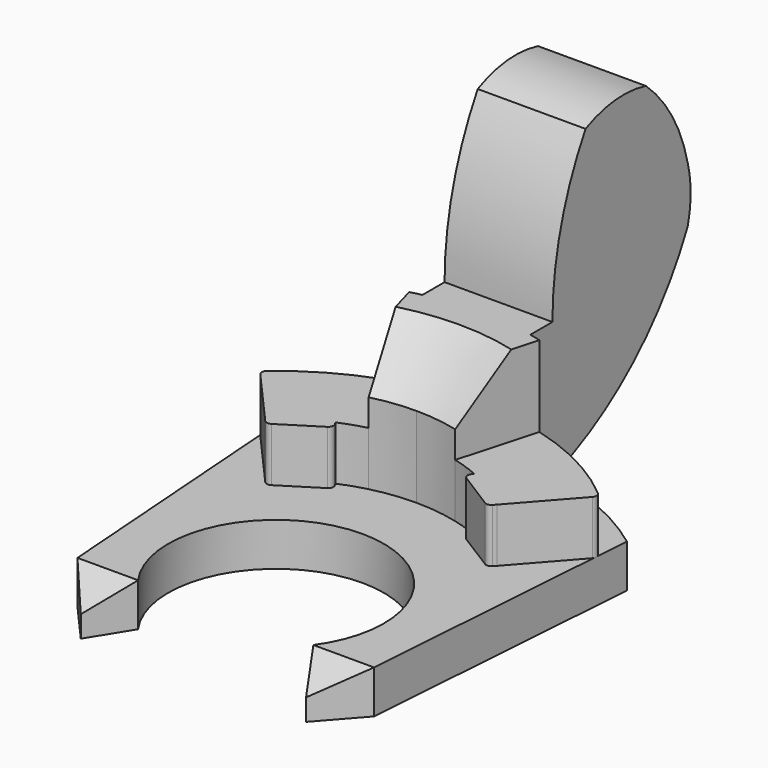
from build123d import *

# Parameters (mm, degrees)
F1_DEPTH      = 1.2
F1_DEPTH_BACK = 0.4
F3_DEPTH      = 12.5
F5_DEPTH      = 2
F6_DEPTH      = 5
F7_T2_ANGLE   = 119.2786087223
F8_DEPTH      = 5
F10_DEPTH     = 4
F11_DEPTH     = 5


# Not quite as in the source:
# - a fillet or chamfer that OpenCascade refuses, or shapes differently, is made with other operations: its cross-section is extruded or revolved along the edge and cut away or added
# - a feature names something its author has since deleted; it is built from what else it names


with BuildPart() as f1:
    # F0 (on Top) → F1 (new body, two sides)
    with BuildSketch(Plane.XY) as f1_sk:
        with BuildLine():
            ThreePointArc((-3.25, -2.3318447633), (0, 4), (3.25, -2.3318447633))
            Line((3.25, -2.3318447633), (4.1771243445, -3.8318447633))
            Line((4.1771243445, -3.8318447633), (5.5, -2.3318447633))
            Line((5.5, -2.3318447633), (6.2861850371, 8.4103434936))
            ThreePointArc((6.2861850371, 8.4103434936), (0, 10.5), (-6.2861850371, 8.4103434936))
            Line((-6.2861850371, 8.4103434936), (-5.5, -2.3318447633))
            Line((-5.5, -2.3318447633), (-4.1771243445, -3.8318447633))
            Line((-4.1771243445, -3.8318447633), (-3.25, -2.3318447633))
        make_face()
    extrude(amount=F1_DEPTH)
    extrude(f1_sk.sketch, amount=-F1_DEPTH_BACK)

    # F2 (on Right) → F3 (cut, symmetric)
    with BuildSketch(Plane.YZ):
        Polygon((-3.8318447633, 0.4), (-2.3318447633, 1.2), (-3.8318447633, 1.2), align=None)
    extrude(amount=F3_DEPTH, both=True, mode=Mode.SUBTRACT)

    # F4 (on face) → F5 (join)
    with BuildSketch(Plane.XY.offset(1.2)):
        with BuildLine():
            Line((0, 9.4893432962), (0, 9.5))
            ThreePointArc((0, 9.5), (-1.0056504861, 9.4466219941), (-2, 9.2870878105))
            ThreePointArc((-2, 9.2870878105), (-2.207287093, 9.2400153511), (-2.4134691055, 9.1883168686))
            Line((-2.4134691055, 9.1883168686), (-1.6054997382, 6.2986006851))
            ThreePointArc((-1.6054997382, 6.2986006851), (-0.809041268, 6.4494536378), (0, 6.5))
            Line((0, 6.5), (0, 9.4893432962))
        make_face()
        with BuildLine():
            Line((0, 10.3126084432), (0, 9.5))
            ThreePointArc((0, 9.5), (1.0056504861, 9.4466219941), (2, 9.2870878105))
            Line((2, 9.2870878105), (2, 10.3126084432))
            Line((2, 10.3126084432), (0, 10.3126084432))
        make_face()
        with BuildLine():
            ThreePointArc((2, 9.2870878105), (1.0056504861, 9.4466219941), (0, 9.5))
            Line((0, 9.5), (0, 9.4893432962))
            Line((0, 9.4893432962), (0, 6.5))
            ThreePointArc((0, 6.5), (0.809041268, 6.4494536378), (1.6054997382, 6.2986006851))
            Line((1.6054997382, 6.2986006851), (2.4134691055, 9.1883168686))
            ThreePointArc((2.4134691055, 9.1883168686), (2.207287093, 9.2400153511), (2, 9.2870878105))
        make_face()
        with BuildLine():
            ThreePointArc((-2, 9.2870878105), (-1.0056504861, 9.4466219941), (0, 9.5))
            Line((0, 9.5), (0, 10.3126084432))
            Line((0, 10.3126084432), (-2, 10.3126084432))
            Line((-2, 10.3126084432), (-2, 9.2870878105))
        make_face()
        with BuildLine():
            Line((-1.6054997382, 6.2986006851), (-2.4134691055, 9.1883168686))
            ThreePointArc((-2.4134691055, 9.1883168686), (-4.3834961594, 8.4282240965), (-6.1369591907, 7.2517399217))
            ThreePointArc((-6.1369591907, 7.2517399217), (-6.2072372931, 7.1135226449), (-6.1576144754, 6.9666192642))
            Line((-6.1576144754, 6.9666192642), (-4.3047045796, 4.8702688306))
            Line((-4.3047045796, 4.8702688306), (-4.2185888433, 4.7728389657))
            ThreePointArc((-4.2185888433, 4.7728389657), (-4.0971505607, 4.7073203992), (-3.9621862374, 4.7360357341))
            Line((-3.9621862374, 4.7360357341), (-2.5827247856, 5.6044208159))
            ThreePointArc((-2.5827247856, 5.6044208159), (-2.4942501859, 5.7293355978), (-2.5200172859, 5.8802246764))
            Line((-2.5200172859, 5.8802246764), (-2.5753119947, 5.968062343))
            ThreePointArc((-2.5753119947, 5.968062343), (-2.096928846, 6.152470188), (-1.6054997382, 6.2986006851))
        make_face()
        with BuildLine():
            ThreePointArc((6.1369591907, 7.2517399217), (4.3834961594, 8.4282240965), (2.4134691055, 9.1883168686))
            Line((2.4134691055, 9.1883168686), (1.6054997382, 6.2986006851))
            ThreePointArc((1.6054997382, 6.2986006851), (2.096928846, 6.152470188), (2.5753119947, 5.968062343))
            Line((2.5753119947, 5.968062343), (2.5200172859, 5.8802246764))
            ThreePointArc((2.5200172859, 5.8802246764), (2.4942501859, 5.7293355978), (2.5827247856, 5.6044208159))
            Line((2.5827247856, 5.6044208159), (3.9621862374, 4.7360357341))
            ThreePointArc((3.9621862374, 4.7360357341), (4.0971505607, 4.7073203992), (4.2185888433, 4.7728389657))
            Line((4.2185888433, 4.7728389657), (4.3047045796, 4.8702688306))
            Line((4.3047045796, 4.8702688306), (6.1576144754, 6.9666192642))
            ThreePointArc((6.1576144754, 6.9666192642), (6.2072372931, 7.1135226449), (6.1369591907, 7.2517399217))
        make_face()
    extrude(amount=F5_DEPTH)

    # F4 (on face) → F6 (join)
    with BuildSketch(Plane.XY.offset(1.2)):
        with BuildLine():
            ThreePointArc((2, 9.2870878105), (1.0056504861, 9.4466219941), (0, 9.5))
            Line((0, 9.5), (0, 9.4893432962))
            Line((0, 9.4893432962), (0, 6.5))
            ThreePointArc((0, 6.5), (0.809041268, 6.4494536378), (1.6054997382, 6.2986006851))
            Line((1.6054997382, 6.2986006851), (2.4134691055, 9.1883168686))
            ThreePointArc((2.4134691055, 9.1883168686), (2.207287093, 9.2400153511), (2, 9.2870878105))
        make_face()
        with BuildLine():
            Line((0, 9.4893432962), (0, 9.5))
            ThreePointArc((0, 9.5), (-1.0056504861, 9.4466219941), (-2, 9.2870878105))
            ThreePointArc((-2, 9.2870878105), (-2.207287093, 9.2400153511), (-2.4134691055, 9.1883168686))
            Line((-2.4134691055, 9.1883168686), (-1.6054997382, 6.2986006851))
            ThreePointArc((-1.6054997382, 6.2986006851), (-0.809041268, 6.4494536378), (0, 6.5))
            Line((0, 6.5), (0, 9.4893432962))
        make_face()
    extrude(amount=F6_DEPTH)

    # F7: chamfer of 2 on 1 edges, made by hand

    # F7_s1 → F7_t2 (revolve, cut)
    with BuildSketch(Plane(origin=(0, 0, 0), x_dir=(0, 0, 1), z_dir=(-0.5054419689, -0.8628606006, 0))):
        Polygon((6.2, 8.5), (4.2, 6.5), (6.2, 6.5), align=None)
    revolve(axis=Axis((0, 0, 6.2), (0, 0, -1)), revolution_arc=F7_T2_ANGLE, mode=Mode.SUBTRACT)

    # F4 (on face) → F8 (join, through all)
    with BuildSketch(Plane.XY.offset(1.2)):
        with BuildLine():
            Line((0, 10.3126084432), (0, 9.5))
            ThreePointArc((0, 9.5), (1.0056504861, 9.4466219941), (2, 9.2870878105))
            Line((2, 9.2870878105), (2, 10.307764064))
            ThreePointArc((2, 10.307764064), (1.9874359165, 10.3101939108), (1.974868881, 10.3126084432))
            Line((1.974868881, 10.3126084432), (0, 10.3126084432))
        make_face()
        with BuildLine():
            ThreePointArc((1.974868881, 10.3126084432), (1.9874359165, 10.3101939108), (2, 10.307764064))
            Line((2, 10.307764064), (2, 10.3126084432))
            Line((2, 10.3126084432), (1.974868881, 10.3126084432))
        make_face()
        with BuildLine():
            Line((-2, 10.3126084432), (-2, 10.307764064))
            ThreePointArc((-2, 10.307764064), (-1.9874359165, 10.3101939108), (-1.974868881, 10.3126084432))
            Line((-1.974868881, 10.3126084432), (-2, 10.3126084432))
        make_face()
        with BuildLine():
            ThreePointArc((-2, 9.2870878105), (-1.0056504861, 9.4466219941), (0, 9.5))
            Line((0, 9.5), (0, 10.3126084432))
            Line((0, 10.3126084432), (-1.974868881, 10.3126084432))
            ThreePointArc((-1.974868881, 10.3126084432), (-1.9874359165, 10.3101939108), (-2, 10.307764064))
            Line((-2, 10.307764064), (-2, 9.2870878105))
        make_face()
    extrude(amount=F8_DEPTH)

    # F9 (on face) → F10 (join)
    with BuildSketch(Plane(origin=(-2, 0, 0), x_dir=(0, -1, 0), z_dir=(-1, 0, 0))):
        with BuildLine():
            Line((-10.4906475171, 1.2), (-10.3126084432, 1.2))
            Line((-10.3126084432, 1.2), (-10.3126084432, 6.2))
            ThreePointArc((-10.3126084432, 6.2), (-10.7033019047, 9.142871965), (-11.848315427, 11.8818646297))
            ThreePointArc((-11.848315427, 11.8818646297), (-13.2228522743, 12.2616673302), (-14.6442650052, 12.1468305588))
            ThreePointArc((-14.6442650052, 12.1468305588), (-15.8696799602, 10.6519801079), (-16.5821556002, 8.8551500812))
            ThreePointArc((-16.5821556002, 8.8551500812), (-16.7217466821, 7.8095628414), (-16.5821556002, 6.7639756016))
            ThreePointArc((-16.5821556002, 6.7639756016), (-14.0870903715, 3.3790869985), (-10.4906475171, 1.2))
        make_face()
    extrude(amount=-F10_DEPTH)

    # F4 (on face) → F11 (join, through all)
    with BuildSketch(Plane.XY.offset(1.2)):
        with BuildLine():
            Line((0, 10.3126084432), (0, 9.5))
            ThreePointArc((0, 9.5), (1.0056504861, 9.4466219941), (2, 9.2870878105))
            Line((2, 9.2870878105), (2, 10.307764064))
            ThreePointArc((2, 10.307764064), (1.9874359165, 10.3101939108), (1.974868881, 10.3126084432))
            Line((1.974868881, 10.3126084432), (0, 10.3126084432))
        make_face()
        with BuildLine():
            ThreePointArc((-2, 9.2870878105), (-1.0056504861, 9.4466219941), (0, 9.5))
            Line((0, 9.5), (0, 10.3126084432))
            Line((0, 10.3126084432), (-1.974868881, 10.3126084432))
            ThreePointArc((-1.974868881, 10.3126084432), (-1.9874359165, 10.3101939108), (-2, 10.307764064))
            Line((-2, 10.307764064), (-2, 9.2870878105))
        make_face()
    extrude(amount=F11_DEPTH)


solid = f1.part
